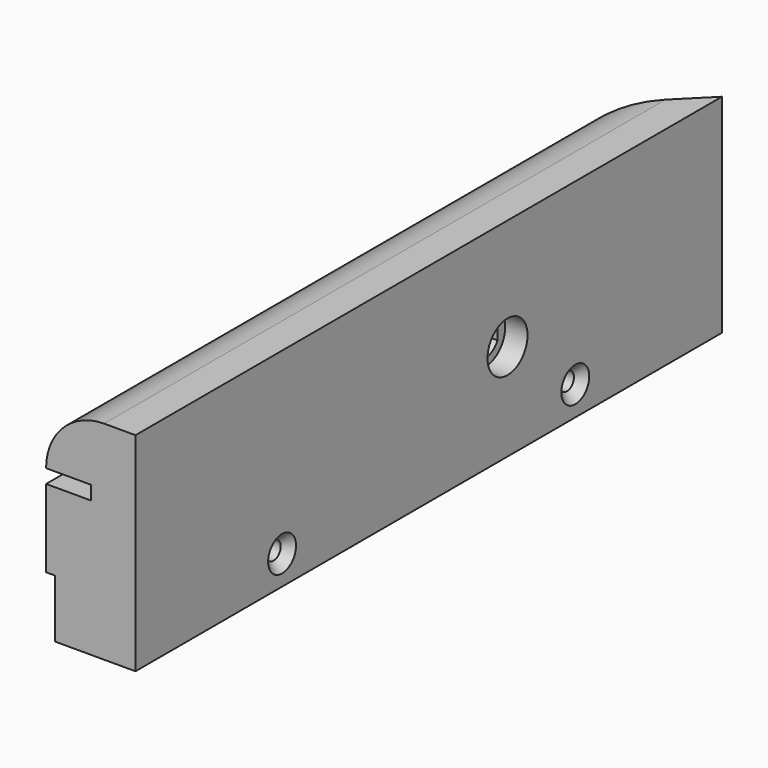
from build123d import *

# Parameters (mm, degrees)
F0_W            = 20
F0_H            = 46.5
F1_DEPTH        = 164
F2_W            = 164
F2_H            = 3.1
F3_DEPTH        = 10
F4_W            = 164
F4_H            = 13
F5_DEPTH        = 2
F7_DEPTH        = 46.5
F8_R            = 12.99999
F10_D           = 4
F10_DEPTH       = 20
F10_CSINK_D     = 7.8
F10_CSINK_ANGLE = 90
F10_TIP         = 1.2017212381
F12_DEPTH       = 20
F13_R           = 7.5
F14_DEPTH       = 13
F15_R           = 5.6
F16_DEPTH       = 5
F17_W           = 38
F17_H           = 15.9
F17_H_2         = 11.1
F18_DEPTH       = 12
F20_DEPTH       = 6
F21_W           = 38
F21_H           = 4
F22_DEPTH       = 4
F23_W           = 38
F23_H           = 4
F24_DEPTH       = 4


# Not quite as in the source:
# - a fillet or chamfer is up to 0.001 mm smaller than in the source, because OpenCascade refuses the exact size


with BuildPart() as f1:
    # F0 (on Front) → F1 (new body)
    with BuildSketch(Plane.XZ):
        Rectangle(F0_W, F0_H)
    extrude(amount=F1_DEPTH)

    # F2 (on face) → F3 (cut)
    with BuildSketch(Plane(origin=(-10, 0, 0), x_dir=(0, -1, 0), z_dir=(-1, 0, 0))):
        with Locations((82, 8.7)):
            Rectangle(F2_W, F2_H)
    extrude(amount=-F3_DEPTH, mode=Mode.SUBTRACT)

    # F4 (on face) → F5 (cut)
    with BuildSketch(Plane(origin=(-10, 0, 0), x_dir=(0, -1, 0), z_dir=(-1, 0, 0))):
        with Locations((82, -16.75)):
            Rectangle(F4_W, F4_H)
    extrude(amount=-F5_DEPTH, mode=Mode.SUBTRACT)

    # F6 (on face) → F7 (cut, through all)
    with BuildSketch(Plane.XY.offset(23.25)):
        Polygon((-10, 0), (-10, -20), (10, 0), align=None)
    extrude(amount=-F7_DEPTH, mode=Mode.SUBTRACT)

    # F8 (radius 13 in the source; OpenCascade refuses exactly that, so slightly less here)
    f8_edges = [f1.edges().sort_by_distance(p)[0] for p in [
        (-10, -92, 23.25),
    ]]
    fillet(f8_edges, radius=F8_R)

    # F10
    with Locations(Plane.YZ.offset(10)):
        with Locations((-123, -16.75), (-41, -16.75)):
            CounterSinkHole(F10_D / 2, F10_CSINK_D / 2, depth=F10_DEPTH, counter_sink_angle=F10_CSINK_ANGLE)
            with Locations((0, 0, -(F10_DEPTH + F10_TIP / 2))):  # 118° drill point
                Cone(0, F10_D / 2, F10_TIP, mode=Mode.SUBTRACT)

    # F11 (on face) → F12 (cut, through all)
    with BuildSketch(Plane(origin=(-10, 0, 0), x_dir=(0, -1, 0), z_dir=(-1, 0, 0))):
        with BuildLine():
            Line((63.4057692308, -3.5508088231), (63.4057692308, 0.4508088231))
            ThreePointArc((63.4057692308, 0.4508088231), (59.9090942784, 2.3989538045), (56.5057692308, 0.2919694165))
            Line((56.5057692308, 0.2919694165), (56.5057692308, -3.3919694165))
            ThreePointArc((56.5057692308, -3.3919694165), (59.9090942784, -5.4989538045), (63.4057692308, -3.5508088231))
        make_face()
    extrude(amount=-F12_DEPTH, mode=Mode.SUBTRACT)

    # F13 (on face) → F14 (cut)
    with BuildSketch(Plane(origin=(-10, 0, 0), x_dir=(0, -1, 0), z_dir=(-1, 0, 0))):
        with Locations((60, -1.55)):
            Circle(F13_R)
        with BuildLine():
            Line((63.4057692308, 0.4508088231), (63.4057692308, -3.5508088231))
            ThreePointArc((63.4057692308, -3.5508088231), (59.9090942784, -5.4989538045), (56.5057692308, -3.3919694165))
            Line((56.5057692308, -3.3919694165), (56.5057692308, 0.2919694165))
            ThreePointArc((56.5057692308, 0.2919694165), (59.9090942784, 2.3989538045), (63.4057692308, 0.4508088231))
        make_face(mode=Mode.SUBTRACT)
    extrude(amount=-F14_DEPTH, mode=Mode.SUBTRACT)

    # F15 (on face) → F16 (cut)
    with BuildSketch(Plane.YZ.offset(10)):
        with Locations((-59.9557692308, -1.6294197033)):
            Circle(F15_R)
        with BuildLine():
            ThreePointArc((-56.5057692308, -3.3919694165), (-59.9090942784, -5.4989538045), (-63.4057692308, -3.5508088231))
            Line((-63.4057692308, -3.5508088231), (-63.4057692308, 0.4508088231))
            ThreePointArc((-63.4057692308, 0.4508088231), (-59.9090942784, 2.3989538045), (-56.5057692308, 0.2919694165))
            Line((-56.5057692308, 0.2919694165), (-56.5057692308, -3.3919694165))
        make_face(mode=Mode.SUBTRACT)
    extrude(amount=-F16_DEPTH, mode=Mode.SUBTRACT)

    # F17 (on face) → F18 (cut)
    with BuildSketch(Plane(origin=(-10, 0, 0), x_dir=(0, -1, 0), z_dir=(-1, 0, 0))):
        with Locations((94, -2.3)):
            Rectangle(F17_W, F17_H)
        with Locations((94, -15.8)):
            Rectangle(F17_W, F17_H_2)
    extrude(amount=-F18_DEPTH, mode=Mode.SUBTRACT)

    # F19 (on face) → F20 (cut)
    with BuildSketch(Plane(origin=(-10, 0, 0), x_dir=(0, -1, 0), z_dir=(-1, 0, 0))):
        with BuildLine():
            Line((75, -3.1), (75, 0))
            Line((75, 0), (67.3380855814, 0))
            ThreePointArc((67.3380855814, 0), (67.4594115673, -0.7707830407), (67.5, -1.55))
            ThreePointArc((67.5, -1.55), (67.4594115673, -2.3292169593), (67.3380855814, -3.1))
            Line((67.3380855814, -3.1), (75, -3.1))
        make_face()
    extrude(amount=-F20_DEPTH, mode=Mode.SUBTRACT)

    # F21 (on face) → F22 (cut)
    with BuildSketch(Plane(origin=(2, 0, 0), x_dir=(0, -1, 0), z_dir=(-1, 0, 0))):
        with Locations((94, 3.65)):
            Rectangle(F21_W, F21_H)
    extrude(amount=-F22_DEPTH, mode=Mode.SUBTRACT)

    # F23 (on face) → F24 (cut)
    with BuildSketch(Plane(origin=(2, 0, 0), x_dir=(0, -1, 0), z_dir=(-1, 0, 0))):
        with Locations((94, -19.35)):
            Rectangle(F23_W, F23_H)
    extrude(amount=-F24_DEPTH, mode=Mode.SUBTRACT)


solid = f1.part
